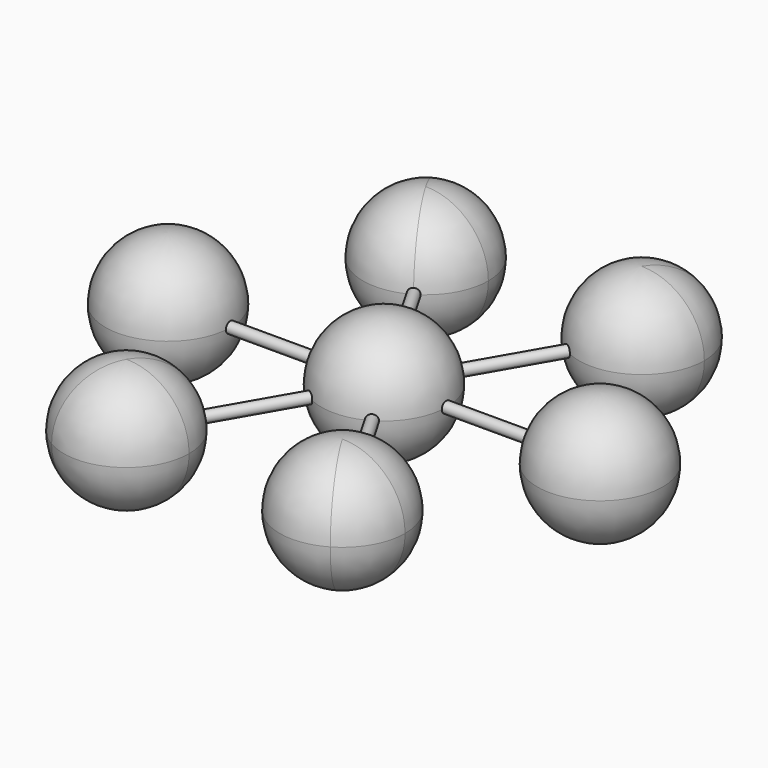
from build123d import *

# Parameters (mm, degrees)
F1_DEPTH = 22.5
F0_R     = 22.5
F2_R     = 22.49999
F2_2_R   = 22.49999
F2_3_R   = 22.49999
F2_4_R   = 22.49999
F2_5_R   = 22.49999
F2_6_R   = 22.49999
F2_7_R   = 22.49999
F5_R     = 2
F8_R     = 2
F11_R    = 2


# Not quite as in the source:
# - a fillet or chamfer is up to 0.001 mm smaller than in the source, because OpenCascade refuses the exact size
# - a feature names something its author has since deleted; it is built from what else it names


with BuildPart() as f1:
    # F0 (on Top) → F1 (new body, symmetric)
    with BuildSketch(Plane.XY):
        with BuildLine():
            ThreePointArc((55, 0), (77.5, -22.5), (100, 0))
            Line((100, 0), (55, 0))
        make_face()
        with BuildLine():
            Line((55, 0), (100, 0))
            ThreePointArc((100, 0), (77.5, 22.5), (55, 0))
        make_face()
    extrude(amount=F1_DEPTH, both=True)

    # F2#5 (radius 22.5 in the source; OpenCascade refuses exactly that, so slightly less here)
    f2_5_edges = [f1.edges().sort_by_distance(p)[0] for p in [
        (55, 0, 22.5),
        (55, 0, -22.5),
    ]]
    fillet(f2_5_edges, radius=F2_5_R)


with BuildPart() as f1b:
    # F0 (on Top) → F1, piece 2 (new body, symmetric)
    with BuildSketch(Plane.XY):
        Circle(F0_R)
    extrude(amount=F1_DEPTH, both=True)

    # F2 (radius 22.5 in the source; OpenCascade refuses exactly that, so slightly less here)
    f2_edges = [f1b.edges().sort_by_distance(p)[0] for p in [
        (-22.5, 0, 22.5),
        (-22.5, 0, -22.5),
    ]]
    fillet(f2_edges, radius=F2_R)


with BuildPart() as f1c:
    # F0 (on Top) → F1, piece 3 (new body, symmetric)
    with BuildSketch(Plane.XY):
        with BuildLine():
            ThreePointArc((61.25, 67.1169687933), (58.2355715851, 78.3669687933), (50, 86.6025403784))
            Line((50, 86.6025403784), (27.5, 47.6313972081))
            ThreePointArc((27.5, 47.6313972081), (50, 47.6313972081), (61.25, 67.1169687933))
        make_face()
        with BuildLine():
            Line((27.5, 47.6313972081), (50, 86.6025403784))
            ThreePointArc((50, 86.6025403784), (19.2644284149, 78.3669687933), (27.5, 47.6313972081))
        make_face()
    extrude(amount=F1_DEPTH, both=True)

    # F2#4 (radius 22.5 in the source; OpenCascade refuses exactly that, so slightly less here)
    f2_4_edges = [f1c.edges().sort_by_distance(p)[0] for p in [
        (16.25, 67.116969, 22.5),
        (16.25, 67.116969, -22.5),
    ]]
    fillet(f2_4_edges, radius=F2_4_R)


with BuildPart() as f1d:
    # F0 (on Top) → F1, piece 4 (new body, symmetric)
    with BuildSketch(Plane.XY):
        with BuildLine():
            ThreePointArc((-16.25, 67.1169687933), (-27.5, 86.6025403784), (-50, 86.6025403784))
            Line((-50, 86.6025403784), (-27.5, 47.6313972081))
            ThreePointArc((-27.5, 47.6313972081), (-19.2644284149, 55.8669687933), (-16.25, 67.1169687933))
        make_face()
        with BuildLine():
            Line((-27.5, 47.6313972081), (-50, 86.6025403784))
            ThreePointArc((-50, 86.6025403784), (-58.2355715851, 55.8669687933), (-27.5, 47.6313972081))
        make_face()
    extrude(amount=F1_DEPTH, both=True)

    # F2#3 (radius 22.5 in the source; OpenCascade refuses exactly that, so slightly less here)
    f2_3_edges = [f1d.edges().sort_by_distance(p)[0] for p in [
        (-61.25, 67.116969, 22.5),
        (-61.25, 67.116969, -22.5),
    ]]
    fillet(f2_3_edges, radius=F2_3_R)


with BuildPart() as f1e:
    # F0 (on Top) → F1, piece 5 (new body, symmetric)
    with BuildSketch(Plane.XY):
        with BuildLine():
            ThreePointArc((27.5, -47.6313972081), (19.2644284149, -78.3669687933), (50, -86.6025403784))
            Line((50, -86.6025403784), (27.5, -47.6313972081))
        make_face()
        with BuildLine():
            Line((27.5, -47.6313972081), (50, -86.6025403784))
            ThreePointArc((50, -86.6025403784), (58.2355715851, -78.3669687933), (61.25, -67.1169687933))
            ThreePointArc((61.25, -67.1169687933), (50, -47.6313972081), (27.5, -47.6313972081))
        make_face()
    extrude(amount=F1_DEPTH, both=True)

    # F2#6 (radius 22.5 in the source; OpenCascade refuses exactly that, so slightly less here)
    f2_6_edges = [f1e.edges().sort_by_distance(p)[0] for p in [
        (27.5, -47.631397, 22.5),
        (27.5, -47.631397, -22.5),
    ]]
    fillet(f2_6_edges, radius=F2_6_R)


with BuildPart() as f1f:
    # F0 (on Top) → F1, piece 6 (new body, symmetric)
    with BuildSketch(Plane.XY):
        with BuildLine():
            ThreePointArc((-27.5, -47.6313972081), (-58.2355715851, -55.8669687933), (-50, -86.6025403784))
            Line((-50, -86.6025403784), (-27.5, -47.6313972081))
        make_face()
        with BuildLine():
            Line((-27.5, -47.6313972081), (-50, -86.6025403784))
            ThreePointArc((-50, -86.6025403784), (-27.5, -86.6025403784), (-16.25, -67.1169687933))
            ThreePointArc((-16.25, -67.1169687933), (-19.2644284149, -55.8669687933), (-27.5, -47.6313972081))
        make_face()
    extrude(amount=F1_DEPTH, both=True)

    # F2#7 (radius 22.5 in the source; OpenCascade refuses exactly that, so slightly less here)
    f2_7_edges = [f1f.edges().sort_by_distance(p)[0] for p in [
        (-27.5, -47.631397, 22.5),
        (-27.5, -47.631397, -22.5),
    ]]
    fillet(f2_7_edges, radius=F2_7_R)


with BuildPart() as f1g:
    # F0 (on Top) → F1, piece 7 (new body, symmetric)
    with BuildSketch(Plane.XY):
        with BuildLine():
            ThreePointArc((-55, 0), (-77.5, 22.5), (-100, 0))
            Line((-100, 0), (-55, 0))
        make_face()
        with BuildLine():
            Line((-55, 0), (-100, 0))
            ThreePointArc((-100, 0), (-77.5, -22.5), (-55, 0))
        make_face()
    extrude(amount=F1_DEPTH, both=True)

    # F2#2 (radius 22.5 in the source; OpenCascade refuses exactly that, so slightly less here)
    f2_2_edges = [f1g.edges().sort_by_distance(p)[0] for p in [
        (-55, 0, 22.5),
        (-55, 0, -22.5),
    ]]
    fillet(f2_2_edges, radius=F2_2_R)


with BuildPart() as f6:
    # F6: sweep along a path in F4
    with BuildLine(Plane.XY) as f6_path:
        Line((-77.5, 0), (77.5, 0))
    # F5 (on offset) → F6 (sweep)
    with BuildSketch(Plane.YZ.offset(79.8)):
        Circle(F5_R)
    sweep(path=f6_path.line)


with BuildPart() as f9:
    # F9: sweep along a path in F4
    with BuildLine(Plane.XY) as f9_path:
        Line((-38.75, 67.1169687933), (38.75, -67.1169687933))
    # F8 (on line) → F9 (sweep)
    with BuildSketch(Plane(origin=(-38.75, 67.1169687933, 0), x_dir=(0.8660254038, 0.5, 0), z_dir=(0.5, -0.8660254038, 0))):
        Circle(F8_R)
    sweep(path=f9_path.line)


with BuildPart() as f12:
    # F12: sweep along a path in F4
    with BuildLine(Plane.XY) as f12_path:
        Line((38.75, 67.1169687933), (-38.75, -67.1169687933))
    # F11 (on line) → F12 (sweep)
    with BuildSketch(Plane(origin=(38.75, 67.1169687933, 0), x_dir=(0.8660254038, -0.5, 0), z_dir=(-0.5, -0.8660254038, 0))):
        Circle(F11_R)
    sweep(path=f12_path.line)


solid = Compound([f1.part, f1b.part, f1c.part, f1d.part, f1e.part, f1f.part, f1g.part, f6.part, f9.part, f12.part])
